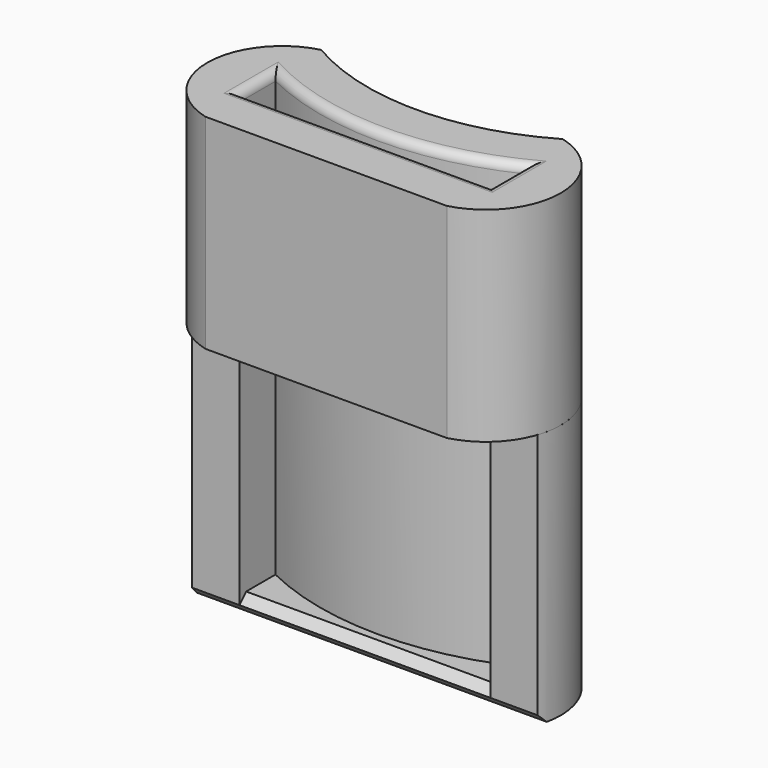
from build123d import *

# Parameters (mm, degrees)
F1_DEPTH = 12
F3_DEPTH = 14
F5_DEPTH = 1
F6_SIZE  = 0.5
F7_SIZE  = 1
F8_SIZE  = 0.49999
F9_R     = 0.5


# Not quite as in the source:
# - a fillet or chamfer is up to 0.001 mm smaller than in the source, because OpenCascade refuses the exact size


with BuildPart() as f1:
    # F0 (on Top) → F1 (new body)
    with BuildSketch(Plane.XY):
        with BuildLine():
            ThreePointArc((2.421303573, 3), (-0.8627873361, -1.25), (2.421303573, -5.5))
            Line((2.421303573, -5.5), (16.6031217548, -5.5))
            ThreePointArc((16.6031217548, -5.5), (19.8872126639, -1.25), (16.6031217548, 3))
            ThreePointArc((16.6031217548, 3), (9.5122126639, 1.0867768062), (2.421303573, 3))
        make_face()
        with BuildLine():
            Line((4.6372126639, -2.65), (2.1372126639, -2.65))
            Line((2.1372126639, -2.65), (2.1372126639, 0))
            ThreePointArc((2.1372126639, 0), (9.5122126639, -1.6934638377), (16.8872126639, 0))
            Line((16.8872126639, 0), (16.8872126639, -2.65))
            Line((16.8872126639, -2.65), (4.6372126639, -2.65))
        make_face(mode=Mode.SUBTRACT)
    extrude(amount=F1_DEPTH)

    # F7
    f7_edges = [f1.edges().sort_by_distance(p)[0] for p in [
        (9.512213, -2.65, 0),
    ]]
    chamfer(f7_edges, length=F7_SIZE)

    # F9
    f9_edges = [f1.edges().sort_by_distance(p)[0] for p in [
        (9.512213, -2.65, 12),
        (2.137213, -1.325, 12),
        (9.512213, -1.693464, 12),
        (16.887213, -1.325, 12),
    ]]
    fillet(f9_edges, radius=F9_R)


with BuildPart() as f3:
    # F2 (on face) → F3 (new body)
    with BuildSketch(Plane(origin=(0, 0, 0), x_dir=(1, 0, 0), z_dir=(0, 0, -1))):
        with BuildLine():
            ThreePointArc((-0.6336811406, 2.65), (-0.3341866365, -0.8389848971), (2.421303573, -3))
            ThreePointArc((2.421303573, -3), (9.5122126639, -1.0867768062), (16.6031217548, -3))
            ThreePointArc((16.6031217548, -3), (19.3586119643, -0.8389848971), (19.6581064684, 2.65))
            Line((19.6581064684, 2.65), (16.8872126639, 2.65))
            Line((16.8872126639, 2.65), (16.8872126639, 0))
            ThreePointArc((16.8872126639, 0), (9.5122126639, 1.6934638377), (2.1372126639, 0))
            Line((2.1372126639, 0), (2.1372126639, 2.65))
            Line((2.1372126639, 2.65), (-0.6336811406, 2.65))
        make_face()
    extrude(amount=F3_DEPTH)

    # F4 (on face) → F5 (join)
    with BuildSketch(Plane(origin=(0, 0, -14), x_dir=(1, 0, 0), z_dir=(0, 0, -1))):
        with BuildLine():
            ThreePointArc((-0.6336811406, 2.65), (-0.3341866365, -0.8389848971), (2.421303573, -3))
            Line((2.421303573, -3), (16.6031217548, -3))
            ThreePointArc((16.6031217548, -3), (19.3586119643, -0.8389848971), (19.6581064684, 2.65))
            Line((19.6581064684, 2.65), (-0.6336811406, 2.65))
        make_face()
    extrude(amount=F5_DEPTH)

    # F6
    f6_edges = [f3.edges().sort_by_distance(p)[0] for p in [
        (9.512213, -2.65, -15),
    ]]
    chamfer(f6_edges, length=F6_SIZE)

    # F8 (size 0.5 in the source; OpenCascade refuses exactly that, so slightly less here)
    f8_edges = [f3.edges().sort_by_distance(p)[0] for p in [
        (9.512213, -2.65, -14),
    ]]
    chamfer(f8_edges, length=F8_SIZE)


solid = Compound([f1.part, f3.part])
